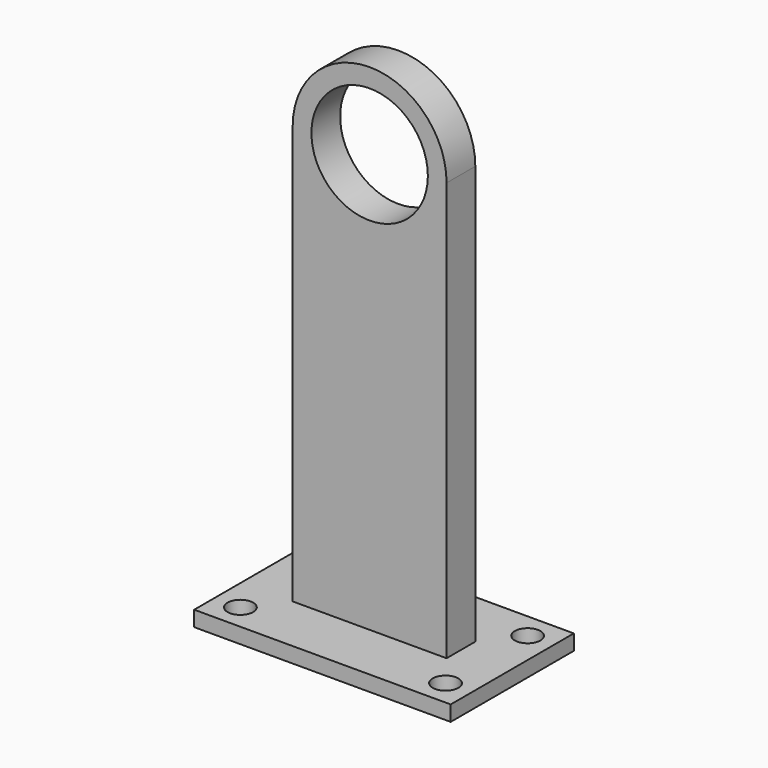
from build123d import *

# Parameters (mm, degrees)
F0_W     = 15
F0_H     = 47
F0_R     = 11.35
F1_DEPTH = 3.5
F2_DEPTH = 15
F3_T     = -3
F4_R     = 2.5
F5_DEPTH = 56


# Not quite as in the source:
# - a shell that OpenCascade refuses in one call is made with other operations: the cavity is built on its own and cut out


with BuildPart() as f1:
    # F0 (on Front) → F1 (new body, symmetric)
    with BuildSketch(Plane.XZ):
        with Locations((7.5, -23.5)):
            Rectangle(F0_W, F0_H)
        with BuildLine():
            Line((0, 0), (15, 0))
            Line((15, 0), (15, 34.5828086023))
            ThreePointArc((15, 34.5828086023), (10.6066017178, 23.9762068845), (0, 19.5828086023))
            Line((0, 19.5828086023), (0, 0))
        make_face()
        with BuildLine():
            ThreePointArc((15, 34.5828086023), (0, 49.5828086023), (-15, 34.5828086023))
            ThreePointArc((-15, 34.5828086023), (-10.6066017178, 23.9762068845), (0, 19.5828086023))
            ThreePointArc((0, 19.5828086023), (10.6066017178, 23.9762068845), (15, 34.5828086023))
        make_face()
        with Locations((0, 34.5828086023)):
            Circle(F0_R, mode=Mode.SUBTRACT)
        with BuildLine():
            Line((-15, 34.5828086023), (-15, 0))
            Line((-15, 0), (0, 0))
            Line((0, 0), (0, 19.5828086023))
            ThreePointArc((0, 19.5828086023), (-10.6066017178, 23.9762068845), (-15, 34.5828086023))
        make_face()
        with Locations((-7.5, -23.5)):
            Rectangle(F0_W, F0_H)
    extrude(amount=F1_DEPTH, both=True)

    # F0 (on Front) → F2 (join, symmetric)
    with BuildSketch(Plane.XZ):
        Polygon((-25, -47), (-25, -50), (25, -50), (25, -47), (15, -47), (0, -47), (-15, -47), align=None)
    extrude(amount=F2_DEPTH, both=True)

    # F3: a shell. OpenCascade refuses it in one call, so the cavity is built on its own and cut out:
    # the body offset inwards by the wall thickness, plus a prism from it out through each open face.
    f3_core = offset(f1.part, amount=F3_T, kind=Kind.INTERSECTION, mode=Mode.PRIVATE)
    f3_exits = [f3_core.faces().sort_by_distance(p)[0] for p in [
        (0, 0.5, -12.400343),
    ]]
    add(f3_core, mode=Mode.SUBTRACT)
    extrude(f3_exits, amount=-F3_T, mode=Mode.SUBTRACT)

    # F4 (on Top) → F5 (cut)
    with BuildSketch(Plane.XY):
        with Locations((20, 10)):
            Circle(F4_R)
        with Locations((-20, 10)):
            Circle(F4_R)
        with Locations((-20, -10)):
            Circle(F4_R)
        with Locations((20, -10)):
            Circle(F4_R)
    extrude(amount=-F5_DEPTH, mode=Mode.SUBTRACT)


solid = f1.part
